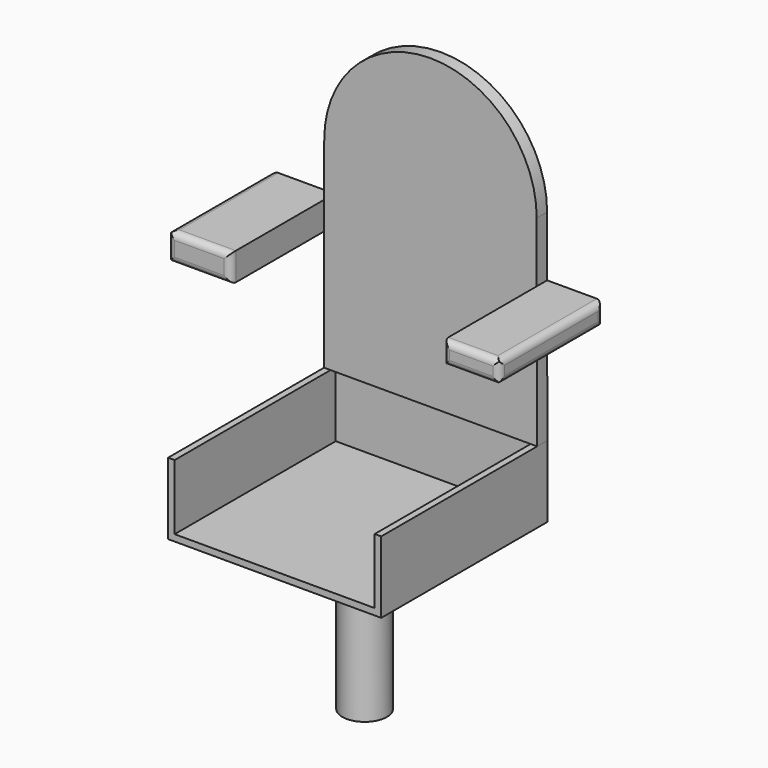
from build123d import *

# Parameters (mm, degrees)
F1_DEPTH     = 25.4
F2_W         = 122.9124367237
F2_H         = 54.4548928738
F2_W_2       = 109.6877083182
F2_H_2       = 43.1749299169
F3_DEPTH     = 25.4
F4_DEPTH     = 254
F5_W         = 416.5798053145
F5_H         = 140.2521133423
F6_DEPTH     = 406.4
F7_T         = 12.7
F7_T3_DEPTH  = 50.8
F7_T5_DEPTH  = 79.8548928738
F7_T7_DEPTH  = 68.5749299169
F9_DEPTH     = 50.8
F10_R        = 43.4523087169
F11_DEPTH    = 261.62
F12_R        = 12.7
F13_R        = 12.7
F14_T1_DEPTH = 304.8
F14_T3_DEPTH = 106.6749299169
F15_T1_DEPTH = 304.8
F15_T3_DEPTH = 117.9548928738


# Not quite as in the source:
# - a fillet or chamfer that OpenCascade refuses, or shapes differently, is made with other operations: its cross-section is extruded or revolved along the edge and cut away or added
# - a shell that OpenCascade refuses in one call is made with other operations: the cavity is built on its own and cut out


with BuildPart() as f1:
    # F0 (on Front) → F1 (new body)
    with BuildSketch(Plane.XZ):
        with BuildLine():
            Line((-327.2927701473, 391.1513090134), (-327.2927701473, 156.2174260616))
            Line((-327.2927701473, 156.2174260616), (-327.2927701473, 0))
            Line((-327.2927701473, 0), (88.8980552554, 0))
            Line((88.8980552554, 0), (88.1201252341, 157.773271203))
            Line((88.1201252341, 157.773271203), (88.1201252341, 392.7071690559))
            ThreePointArc((88.1201252341, 392.7071690559), (-120.3671715418, 600.4150735454), (-327.2927701473, 391.1513090134))
        make_face()
    extrude(amount=F1_DEPTH)

    # F2 (on Front) → F3 (join)
    with BuildSketch(Plane.XZ):
        with Locations((-388.7489885092, 262.0154768229)):
            Rectangle(F2_W, F2_H)
        with Locations((142.9639793932, 253.6527551711)):
            Rectangle(F2_W_2, F2_H_2)
    extrude(amount=F3_DEPTH)

    # F2 (on Front) → F4 (join)
    with BuildSketch(Plane.XZ):
        with Locations((142.9639793932, 253.6527551711)):
            Rectangle(F2_W_2, F2_H_2)
        with Locations((-388.7489885092, 262.0154768229)):
            Rectangle(F2_W, F2_H)
    extrude(amount=F4_DEPTH)

    # F5 (on Front) → F6 (join)
    with BuildSketch(Plane.XZ):
        with Locations((-119.3918474019, -70.1260566711)):
            Rectangle(F5_W, F5_H)
    extrude(amount=F6_DEPTH)

    # F7: shell of thickness 12.7, made by hand


with BuildPart() as f7_core1:
    # F7_t2: copy of F1
    add(f1.part)

    # the walls: a layer under each face that stays
    f7_faces = [f7_core1.faces().sort_by_distance(p)[0] for p in [
        (-327.2927701473, -12.7, 340.1971161366),
        (-126.1986866593, 0, 230.0822085061),
        (-388.7489885092, -127, 289.2429232597),
        (-119.2002710537, -25.4, 300.2082651772),
        (-120.3671715418, -12.7, 600.4150735454),
        (-450.205206871, -127, 262.0154768229),
        (-388.7489885092, -127, 234.788030386),
        (-327.2927701473, -12.7, 117.394015193),
        (88.5090902448, -12.7, 78.8866356015),
        (88.1201252341, -12.7, 194.9192807078),
        (142.9639793932, -127, 232.0652902126),
        (197.8078335524, -127, 253.6527551711),
        (142.9639793932, -127, 275.2402201295),
        (88.1201252341, -12.7, 333.9736945927),
        (-327.2927701473, -139.7, 262.0154768229),
        (-388.7489885092, -254, 262.0154768229),
        (88.1201252341, -139.7, 253.6527551711),
        (-327.6817500591, -203.2, -70.1260566711),
        (-119.3918474019, -203.2, -140.2521133423),
        (88.8980552554, -203.2, -70.1260566711),
        (142.9639793932, -254, 253.6527551711),
    ]]
    thicken(f7_faces, amount=-F7_T, mode=Mode.SUBTRACT)

    # F7_s4 → F7_t3 (cut)
    with BuildSketch(Plane.XZ.offset(-12.7)):
        Polygon((-327.4197701473, 289.3699232597), (-314.5927701473, 289.2429232597), (-314.5927701473, 276.5429232597), (-327.2927701473, 276.5429232597), align=None)
        Polygon((-327.5467665844, 391.1503577119), (-314.5927701473, 391.1513090134), (-314.5927701473, 391.1988747552), (-314.5931264415, 391.2464391626), align=None)
        Polygon((-327.4197701473, 234.661030386), (-327.2927701473, 247.488030386), (-314.5927701473, 247.488030386), (-314.5927701473, 234.788030386), align=None)
        Polygon((88.3741236904, 157.7738973922), (75.4202796102, 157.7106522873), (75.4201252341, 157.7419615549), (75.4201252341, 157.773271203), align=None)
        Polygon((88.2471252341, 231.9382902126), (75.4201252341, 232.0652902126), (75.4201252341, 244.7652902126), (88.1201252341, 244.7652902126), align=None)
        Polygon((88.2471252341, 275.3672201295), (88.1201252341, 262.5402201295), (75.4201252341, 262.5402201295), (75.4201252341, 275.2402201295), align=None)
    extrude(amount=F7_T3_DEPTH, mode=Mode.SUBTRACT)

    # F7_s6 → F7_t5 (cut)
    with BuildSketch(Plane.XY.offset(222.088030386)):
        Polygon((-327.1657701473, -25.527), (-327.2927701473, -12.7), (-339.9927701473, -12.7), (-339.9927701473, -25.4), align=None)
    extrude(amount=F7_T5_DEPTH, mode=Mode.SUBTRACT)

    # F7_s8 → F7_t7 (cut)
    with BuildSketch(Plane.XY.offset(219.3652902126)):
        Polygon((87.9931252341, -25.527), (88.1201252341, -12.7), (100.8201252341, -12.7), (100.8201252341, -25.4), align=None)
    extrude(amount=F7_T7_DEPTH, mode=Mode.SUBTRACT)


with BuildPart() as f1_1:
    add(f1.part)

    # what is left inside the walls is the cavity
    f7_cavity = [f7_core1.part.solids().sort_by_distance(p)[0] for p in [
        (-388.748989, -165.1, 276.415923),
        (142.963979, -165.1, 244.89229),
        (-119.391847, -275.166667, -127.425113),
    ]]
    add(f7_cavity, mode=Mode.SUBTRACT)

    # F8 (on face) → F9 (join)
    with BuildSketch(Plane(origin=(0, 0, -140.2521133423), x_dir=(1, 0, 0), z_dir=(0, 0, -1))):
        with BuildLine():
            add(Edge.make_bspline(
                [(23.5522184521, 188.2828474045), (23.5522184521, 313.2291982087), (-188.821808435, 250.7560228066), (-401.1958353221, 188.2828474045), (-188.821808435, 125.8096720023), (23.5522184521, 63.3364966002), (23.5522184521, 188.2828474045)],
                knots=[0, 0, 0, 2.0943951024, 2.0943951024, 4.1887902048, 4.1887902048, 6.2831853072, 6.2831853072, 6.2831853072], degree=2, weights=[1, 0.5, 1, 0.5, 1, 0.5, 1]))
        make_face()
    extrude(amount=F9_DEPTH)

    # F10 (on face) → F11 (join)
    with BuildSketch(Plane(origin=(0, 0, -191.0521133423), x_dir=(1, 0, 0), z_dir=(0, 0, -1))):
        with Locations((-118.0304661393, 188.2828474045)):
            Circle(F10_R)
    extrude(amount=F11_DEPTH)

    # F12
    f12_edges = [f1_1.edges().sort_by_distance(p)[0] for p in [
        (142.963979, -254, 275.24022),
        (88.120125, -254, 253.652755),
        (142.963979, -254, 232.06529),
        (197.807834, -254, 253.652755),
    ]]
    fillet(f12_edges, radius=F12_R)

    # F13
    f13_edges = [f1_1.edges().sort_by_distance(p)[0] for p in [
        (-327.29277, -254, 262.015477),
        (-388.748989, -254, 289.242923),
        (-450.205207, -254, 262.015477),
        (-388.748989, -254, 234.78803),
    ]]
    fillet(f13_edges, radius=F13_R)

    # F14: fillet of radius 12.7 on 4 edges, made by hand

    # F14_s2 → F14_t1 (cut)
    with BuildSketch(Plane.XZ.offset(-31.75)):
        with BuildLine():
            ThreePointArc((185.1078335524, 232.0652902126), (194.0880896734, 235.7850340916), (197.8078335524, 244.7652902126))
            Line((197.8078335524, 244.7652902126), (197.8078335524, 232.0652902126))
            Line((197.8078335524, 232.0652902126), (185.1078335524, 232.0652902126))
        make_face()
        with BuildLine():
            ThreePointArc((197.8078335524, 262.5402201295), (194.0880896734, 271.5204762506), (185.1078335524, 275.2402201295))
            Line((185.1078335524, 275.2402201295), (197.8078335524, 275.2402201295))
            Line((197.8078335524, 275.2402201295), (197.8078335524, 262.5402201295))
        make_face()
    extrude(amount=F14_T1_DEPTH, mode=Mode.SUBTRACT)

    # F14_s4 → F14_t3 (cut)
    with BuildSketch(Plane.XY.offset(200.3152902126)):
        with BuildLine():
            ThreePointArc((185.1078335524, 0), (194.0880896734, -3.7197438789), (197.8078335524, -12.7))
            Line((197.8078335524, -12.7), (197.8078335524, 0))
            Line((197.8078335524, 0), (185.1078335524, 0))
        make_face()
    extrude(amount=F14_T3_DEPTH, mode=Mode.SUBTRACT)

    # F15: fillet of radius 12.7 on 4 edges, made by hand

    # F15_s2 → F15_t1 (cut)
    with BuildSketch(Plane.XZ.offset(-31.75)):
        with BuildLine():
            ThreePointArc((-437.505206871, 289.2429232597), (-446.4854629921, 285.5231793808), (-450.205206871, 276.5429232597))
            Line((-450.205206871, 276.5429232597), (-450.459206871, 276.5429232597))
            Line((-450.459206871, 276.5429232597), (-450.459206871, 289.4969232597))
            Line((-450.459206871, 289.4969232597), (-437.505206871, 289.4969232597))
            Line((-437.505206871, 289.4969232597), (-437.505206871, 289.2429232597))
        make_face()
        with BuildLine():
            ThreePointArc((-450.205206871, 247.488030386), (-446.4854629921, 238.5077742649), (-437.505206871, 234.788030386))
            Line((-437.505206871, 234.788030386), (-437.505206871, 234.534030386))
            Line((-437.505206871, 234.534030386), (-450.459206871, 234.534030386))
            Line((-450.459206871, 234.534030386), (-450.459206871, 247.488030386))
            Line((-450.459206871, 247.488030386), (-450.205206871, 247.488030386))
        make_face()
    extrude(amount=F15_T1_DEPTH, mode=Mode.SUBTRACT)

    # F15_s4 → F15_t3 (cut)
    with BuildSketch(Plane.XY.offset(203.038030386)):
        with BuildLine():
            ThreePointArc((-450.205206871, -12.7), (-446.4854629921, -3.7197438789), (-437.505206871, 0))
            Line((-437.505206871, 0), (-437.505206871, 0.254))
            Line((-437.505206871, 0.254), (-450.459206871, 0.254))
            Line((-450.459206871, 0.254), (-450.459206871, -12.7))
            Line((-450.459206871, -12.7), (-450.205206871, -12.7))
        make_face()
    extrude(amount=F15_T3_DEPTH, mode=Mode.SUBTRACT)


solid = f1_1.part
